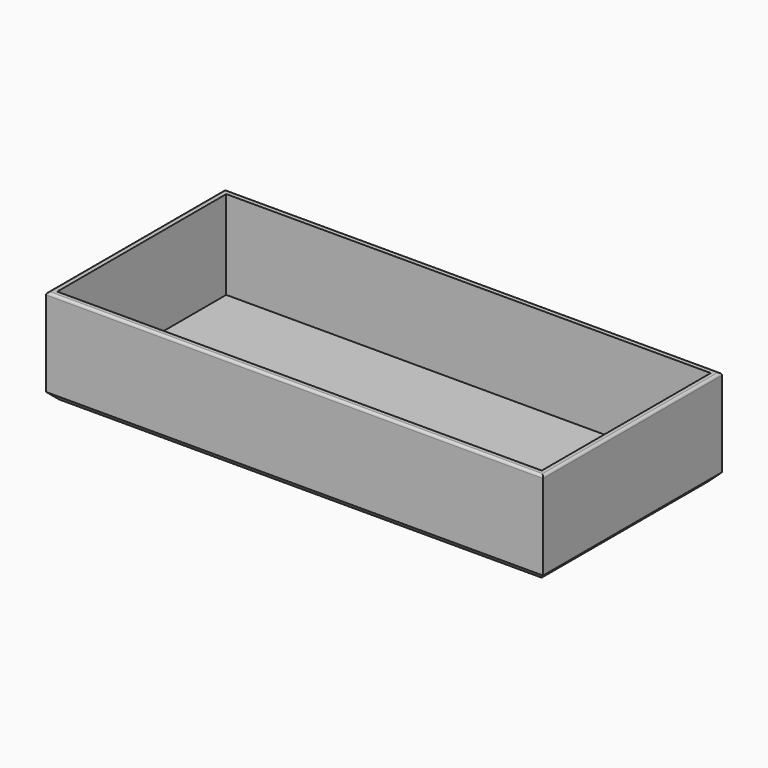
from build123d import *

# Parameters (mm, degrees)
F0_W     = 140
F0_H     = 63
F1_DEPTH = 1.75
F2_W     = 140
F2_H     = 63
F2_W_2   = 136.5
F2_H_2   = 59.5
F3_DEPTH = 25
F4_R     = 0.7
F5_SIZE  = 2


with BuildPart() as f1:
    # F0 (on Top) → F1 (new body)
    with BuildSketch(Plane.XY):
        with Locations((2.7499999851, -32.9423031422)):
            Rectangle(F0_W, F0_H)
    extrude(amount=F1_DEPTH)

    # F2 (on face) → F3 (join)
    with BuildSketch(Plane.XY.offset(1.75)):
        with Locations((2.7499999851, -32.9423031422)):
            Rectangle(F2_W, F2_H)
        with Locations((2.7499999851, -32.9423031422)):
            Rectangle(F2_W_2, F2_H_2, mode=Mode.SUBTRACT)
    extrude(amount=F3_DEPTH)

    # F4
    f4_edges = [f1.edges().sort_by_distance(p)[0] for p in [
        (2.75, -1.442303, 26.75),
        (72.75, -32.942303, 26.75),
        (2.75, -64.442303, 26.75),
        (-67.25, -32.942303, 26.75),
    ]]
    fillet(f4_edges, radius=F4_R)

    # F5
    f5_edges = [f1.edges().sort_by_distance(p)[0] for p in [
        (2.75, -1.442303, 0),
        (-67.25, -32.942303, 0),
        (2.75, -64.442303, 0),
        (72.75, -32.942303, 0),
    ]]
    chamfer(f5_edges, length=F5_SIZE)


solid = f1.part
